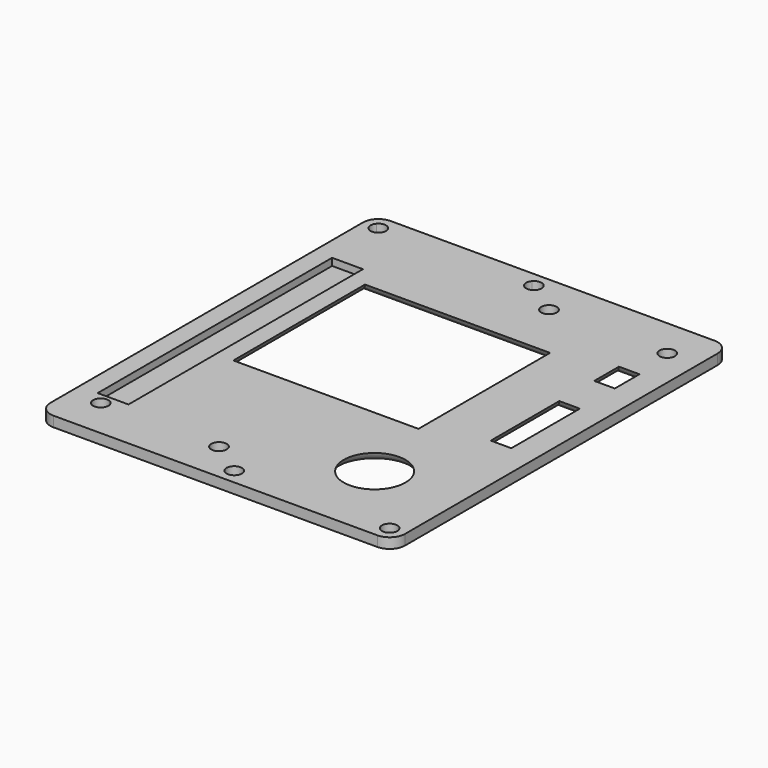
from build123d import *

# Parameters (mm, degrees)
F0_R          = 1.5
F0_R_2        = 6
F0_W          = 6
F0_H          = 57
F0_W_2        = 36
F0_H_2        = 32
F0_W_3        = 4
F0_H_3        = 16.6644380502
F0_H_4        = 6
F0_W_4        = 4.7
F0_H_5        = 2
F0_W_5        = 13
F0_W_6        = 2.3
F0_W_7        = 1.5
F0_W_8        = 9
F0_W_9        = 11
F1_DEPTH      = 2
F2_T1_DEPTH   = 16.6644380502
F2_T3_DEPTH   = 4
F2_T5_DEPTH   = 6
F2_T7_DEPTH   = 32
F2_T9_DEPTH   = 36
F2_T17_DEPTH  = 11.0710678119
F2_T21_DEPTH  = 23.7355058621
F2_T28_DEPTH  = 11.0710678119
F2_T32_DEPTH  = 23.7355058621
F2_T39_DEPTH  = 23.7355058621
F2_T43_DEPTH  = 11.0710678119
F2_T51_DEPTH  = 11.0710678119
F2_T56_DEPTH  = 23.7355058621
F2_T63_DEPTH  = 13.0710678119
F2_T67_DEPTH  = 11.0710678119
F2_T75_DEPTH  = 13.0710678119
F2_T79_DEPTH  = 11.0710678119
F2_T86_DEPTH  = 11.0710678119
F2_T91_DEPTH  = 13.0710678119
F2_S93_R      = 1.5
F2_T94_DEPTH  = 8
F2_T100_DEPTH = 13.0710678119
F2_T104_DEPTH = 11.0710678119
F2_T111_DEPTH = 43.0710678119
F2_T115_DEPTH = 39.0710678119
F2_T122_DEPTH = 39.0710678119
F2_T126_DEPTH = 43.0710678119
F2_T133_DEPTH = 39.0710678119
F2_T137_DEPTH = 43.0710678119
F2_T145_DEPTH = 39.0710678119
F2_T149_DEPTH = 43.0710678119
F3_R          = 3
F4_DEPTH      = 0.6


# Not quite as in the source:
# - a fillet or chamfer that OpenCascade refuses, or shapes differently, is made with other operations: its cross-section is extruded or revolved along the edge and cut away or added


with BuildPart() as f1:
    # F0 (on Top) → F1 (new body)
    with BuildSketch(Plane.XY):
        with BuildLine():
            Line((12.5, -41), (34.5, -41))
            Line((34.5, -41), (34.5, 39))
            Line((34.5, 39), (28.5, 39))
            Line((28.5, 39), (25.5, 39))
            Line((25.5, 39), (20.8, 39))
            Line((20.8, 39), (7.8, 39))
            Line((7.8, 39), (5.5, 39))
            Line((5.5, 39), (-0.1319660113, 39))
            ThreePointArc((-0.1319660113, 39), (0.1512585384, 38.5352331347), (0.25, 38))
            ThreePointArc((0.25, 38), (-1.7852331347, 36.5987414616), (-2.3680339887, 39))
            Line((-2.3680339887, 39), (-5.5, 39))
            Line((-5.5, 39), (-14.5, 39))
            Line((-14.5, 39), (-25.5, 39))
            Line((-25.5, 39), (-27, 39))
            Line((-27, 39), (-28.5, 39))
            Line((-28.5, 39), (-30.3819660113, 39))
            ThreePointArc((-30.3819660113, 39), (-30.0987414616, 38.5352331347), (-30, 38))
            ThreePointArc((-30, 38), (-32.0352331347, 36.5987414616), (-32.6180339887, 39))
            Line((-32.6180339887, 39), (-34.5, 39))
            Line((-34.5, 39), (-34.5, -41))
            Line((-34.5, -41), (-12.5, -41))
            Line((-12.5, -41), (-10.5, -41))
            Line((-10.5, -41), (10.5, -41))
            Line((10.5, -41), (12.5, -41))
        make_face()
        with Locations((-28.5, -33.25)):
            Circle(F0_R, mode=Mode.SUBTRACT)
        with Locations((-5.5, -33.25)):
            Circle(F0_R, mode=Mode.SUBTRACT)
        with Locations((1.25, -38)):
            Circle(F0_R, mode=Mode.SUBTRACT)
        with Locations((31.5, -38)):
            Circle(F0_R, mode=Mode.SUBTRACT)
        with Locations((18, -24.7891994715)):
            Circle(F0_R_2, mode=Mode.SUBTRACT)
        with Locations((-27.9, -2.5)):
            Rectangle(F0_W, F0_H, mode=Mode.SUBTRACT)
        with Locations((-3.5, 6.25)):
            Rectangle(F0_W_2, F0_H_2, mode=Mode.SUBTRACT)
        with Locations((-28.5, 33.25)):
            Circle(F0_R, mode=Mode.SUBTRACT)
        with Locations((-5.5, 33.25)):
            Circle(F0_R, mode=Mode.SUBTRACT)
        with Locations((27.5, 2.4177809749)):
            Rectangle(F0_W_3, F0_H_3, mode=Mode.SUBTRACT)
        with Locations((5.5, 33.25)):
            Circle(F0_R, mode=Mode.SUBTRACT)
        with Locations((27.5, 22.25)):
            Rectangle(F0_W_3, F0_H_4, mode=Mode.SUBTRACT)
        with Locations((28.5, 33.25)):
            Circle(F0_R, mode=Mode.SUBTRACT)
        Polygon((28.5, 39), (34.5, 39), (34.5, 41), (28, 41), (25.5, 41), (25.5, 39), align=None)
        with Locations((23.15, 40)):
            Rectangle(F0_W_4, F0_H_5)
        with Locations((14.3, 40)):
            Rectangle(F0_W_5, F0_H_5)
        with Locations((6.65, 40)):
            Rectangle(F0_W_6, F0_H_5)
        with BuildLine():
            Line((-34.5, 41), (-34.5, 39))
            Line((-34.5, 39), (-32.6180339887, 39))
            ThreePointArc((-32.6180339887, 39), (-31.5, 39.5), (-30.3819660113, 39))
            Line((-30.3819660113, 39), (-28.5, 39))
            Line((-28.5, 39), (-27, 39))
            Line((-27, 39), (-27, 41))
            Line((-27, 41), (-34.5, 41))
        make_face()
        with BuildLine():
            Line((-0.1319660113, 39), (5.5, 39))
            Line((5.5, 39), (5.5, 41))
            Line((5.5, 41), (-5.5, 41))
            Line((-5.5, 41), (-5.5, 39))
            Line((-5.5, 39), (-2.3680339887, 39))
            ThreePointArc((-2.3680339887, 39), (-1.25, 39.5), (-0.1319660113, 39))
        make_face()
        with Locations((-26.25, 40)):
            Rectangle(F0_W_7, F0_H_5)
        with Locations((-10, 40)):
            Rectangle(F0_W_8, F0_H_5)
        with Locations((-20, 40)):
            Rectangle(F0_W_9, F0_H_5)
        with Locations((-28.5, 33.25)):
            Circle(F0_R)
        with Locations((-5.5, 33.25)):
            Circle(F0_R)
    extrude(amount=F1_DEPTH)

    # F2: fillet of radius 3 on 13 edges, made by hand

    # F2_s2 → F2_t1 (cut)
    with BuildSketch(Plane.XZ.offset(-10.75)):
        with BuildLine():
            ThreePointArc((25.5, 2), (24.4036236828, 0.5505102572), (22.6715728753, 0))
            Line((22.6715728753, 0), (25.5, 0))
            Line((25.5, 0), (25.5, 2))
        make_face()
        with BuildLine():
            ThreePointArc((29.5, 2), (30.5963763172, 0.5505102572), (32.3284271247, 0))
            Line((32.3284271247, 0), (29.5, 0))
            Line((29.5, 0), (29.5, 2))
        make_face()
    extrude(amount=F2_T1_DEPTH, mode=Mode.SUBTRACT)

    # F2_s4 → F2_t3 (cut)
    with BuildSketch(Plane.YZ.offset(25.5)):
        with BuildLine():
            ThreePointArc((-5.9144380502, 2), (-7.0108143674, 0.5505102572), (-8.742865175, 0))
            Line((-8.742865175, 0), (-5.9144380502, 0))
            Line((-5.9144380502, 0), (-5.9144380502, 2))
        make_face()
        with BuildLine():
            ThreePointArc((10.75, 2), (11.8463763172, 0.5505102572), (13.5784271247, 0))
            Line((13.5784271247, 0), (10.75, 0))
            Line((10.75, 0), (10.75, 2))
        make_face()
        with BuildLine():
            ThreePointArc((19.25, 2), (18.1536236828, 0.5505102572), (16.4215728753, 0))
            Line((16.4215728753, 0), (19.25, 0))
            Line((19.25, 0), (19.25, 2))
        make_face()
        with BuildLine():
            ThreePointArc((25.25, 2), (26.3463763172, 0.5505102572), (28.0784271247, 0))
            Line((28.0784271247, 0), (25.25, 0))
            Line((25.25, 0), (25.25, 2))
        make_face()
    extrude(amount=F2_T3_DEPTH, mode=Mode.SUBTRACT)

    # F2_s6 → F2_t5 (cut)
    with BuildSketch(Plane.XZ.offset(-25.25)):
        with BuildLine():
            ThreePointArc((29.5, 2), (30.5963763172, 0.5505102572), (32.3284271247, 0))
            Line((32.3284271247, 0), (29.5, 0))
            Line((29.5, 0), (29.5, 2))
        make_face()
        with BuildLine():
            ThreePointArc((25.5, 2), (24.4036236828, 0.5505102572), (22.6715728753, 0))
            Line((22.6715728753, 0), (25.5, 0))
            Line((25.5, 0), (25.5, 2))
        make_face()
    extrude(amount=F2_T5_DEPTH, mode=Mode.SUBTRACT)

    # F2_s8 → F2_t7 (cut)
    with BuildSketch(Plane.XZ.offset(-22.25)):
        with BuildLine():
            ThreePointArc((14.5, 2), (15.5963763172, 0.5505102572), (17.3284271247, 0))
            Line((17.3284271247, 0), (14.5, 0))
            Line((14.5, 0), (14.5, 2))
        make_face()
        with BuildLine():
            ThreePointArc((-21.5, 2), (-22.5963763172, 0.5505102572), (-24.3284271247, 0))
            Line((-24.3284271247, 0), (-21.5, 0))
            Line((-21.5, 0), (-21.5, 2))
        make_face()
    extrude(amount=F2_T7_DEPTH, mode=Mode.SUBTRACT)

    # F2_s10 → F2_t9 (cut)
    with BuildSketch(Plane.YZ.offset(-21.5)):
        with BuildLine():
            ThreePointArc((-9.75, 2), (-10.8463763172, 0.5505102572), (-12.5784271247, 0))
            Line((-12.5784271247, 0), (-9.75, 0))
            Line((-9.75, 0), (-9.75, 2))
        make_face()
        with BuildLine():
            ThreePointArc((22.25, 2), (23.3463763172, 0.5505102572), (25.0784271247, 0))
            Line((25.0784271247, 0), (22.25, 0))
            Line((22.25, 0), (22.25, 2))
        make_face()
    extrude(amount=F2_T9_DEPTH, mode=Mode.SUBTRACT)

    # F2_s11 → F2_t12 (revolve, cut)
    with BuildSketch(Plane.XZ.offset(24.7891994715)):
        with BuildLine():
            ThreePointArc((24, 2), (25.0963763172, 0.5505102572), (26.8284271247, 0))
            Line((26.8284271247, 0), (24, 0))
            Line((24, 0), (24, 2))
        make_face()
    revolve(axis=Axis((18, -24.7891994715, 0), (0, 0, 1)), mode=Mode.SUBTRACT)


with BuildPart() as f2_tool15:
    # F2_s16 → F2_t17 (new body)
    with BuildSketch(Plane.YZ.offset(29.5)):
        with BuildLine():
            ThreePointArc((-5.9144380502, 2), (-7.0108143674, 0.5505102572), (-8.742865175, 0))
            Line((-8.742865175, 0), (-5.9144380502, 0))
            Line((-5.9144380502, 0), (-5.9144380502, 2))
        make_face()
    extrude(amount=-F2_T17_DEPTH)

    split(bisect_by=Plane.YZ.offset(25.5), keep=Keep.BOTTOM)


with BuildPart() as f2_tool19:
    # F2_s20 → F2_t21 (new body)
    with BuildSketch(Plane.XZ.offset(12.9855058621)):
        with BuildLine():
            ThreePointArc((25.5, 2), (24.4036236828, 0.5505102572), (22.6715728753, 0))
            Line((22.6715728753, 0), (25.5, 0))
            Line((25.5, 0), (25.5, 2))
        make_face()
    extrude(amount=-F2_T21_DEPTH)

    split(bisect_by=Plane.XZ.offset(5.9144380502), keep=Keep.TOP)


with BuildPart() as f2_tool15_1:
    add(f2_tool15.part)

    # F2_t23: intersect F2_tool19
    add(f2_tool19.part, mode=Mode.INTERSECT)


with BuildPart() as f1_1:
    add(f1.part)

    # F2_t13: cut F2_tool15
    add(f2_tool15_1.part, mode=Mode.SUBTRACT)


with BuildPart() as f2_tool26:
    # F2_s27 → F2_t28 (new body)
    with BuildSketch(Plane.YZ.offset(18.4289321881)):
        with BuildLine():
            ThreePointArc((10.75, 2), (11.8463763172, 0.5505102572), (13.5784271247, 0))
            Line((13.5784271247, 0), (10.75, 0))
            Line((10.75, 0), (10.75, 2))
        make_face()
    extrude(amount=F2_T28_DEPTH)

    split(bisect_by=Plane.YZ.offset(25.5), keep=Keep.BOTTOM)


with BuildPart() as f2_tool30:
    # F2_s31 → F2_t32 (new body)
    with BuildSketch(Plane.XZ.offset(5.9144380502)):
        with BuildLine():
            ThreePointArc((25.5, 2), (24.4036236828, 0.5505102572), (22.6715728753, 0))
            Line((22.6715728753, 0), (25.5, 0))
            Line((25.5, 0), (25.5, 2))
        make_face()
    extrude(amount=-F2_T32_DEPTH)

    split(bisect_by=Plane.XZ.offset(-10.75), keep=Keep.BOTTOM)


with BuildPart() as f2_tool26_1:
    add(f2_tool26.part)

    # F2_t34: intersect F2_tool30
    add(f2_tool30.part, mode=Mode.INTERSECT)


with BuildPart() as f1_2:
    add(f1_1.part)

    # F2_t24: cut F2_tool26
    add(f2_tool26_1.part, mode=Mode.SUBTRACT)


with BuildPart() as f2_tool37:
    # F2_s38 → F2_t39 (new body)
    with BuildSketch(Plane.XZ.offset(-10.75)):
        with BuildLine():
            ThreePointArc((29.5, 2), (30.5963763172, 0.5505102572), (32.3284271247, 0))
            Line((32.3284271247, 0), (29.5, 0))
            Line((29.5, 0), (29.5, 2))
        make_face()
    extrude(amount=F2_T39_DEPTH)

    split(bisect_by=Plane.XZ.offset(5.9144380502), keep=Keep.TOP)


with BuildPart() as f2_tool41:
    # F2_s42 → F2_t43 (new body)
    with BuildSketch(Plane.YZ.offset(36.5710678119)):
        with BuildLine():
            ThreePointArc((-5.9144380502, 2), (-7.0108143674, 0.5505102572), (-8.742865175, 0))
            Line((-8.742865175, 0), (-5.9144380502, 0))
            Line((-5.9144380502, 0), (-5.9144380502, 2))
        make_face()
    extrude(amount=-F2_T43_DEPTH)

    split(bisect_by=Plane.YZ.offset(34.5), keep=Keep.BOTTOM)

    split(bisect_by=Plane.YZ.offset(29.5), keep=Keep.TOP)


with BuildPart() as f2_tool37_1:
    add(f2_tool37.part)

    # F2_t46: intersect F2_tool41
    add(f2_tool41.part, mode=Mode.INTERSECT)


with BuildPart() as f1_3:
    add(f1_2.part)

    # F2_t35: cut F2_tool37
    add(f2_tool37_1.part, mode=Mode.SUBTRACT)


with BuildPart() as f2_tool49:
    # F2_s50 → F2_t51 (new body)
    with BuildSketch(Plane.YZ.offset(25.5)):
        with BuildLine():
            ThreePointArc((10.75, 2), (11.8463763172, 0.5505102572), (13.5784271247, 0))
            Line((13.5784271247, 0), (10.75, 0))
            Line((10.75, 0), (10.75, 2))
        make_face()
    extrude(amount=F2_T51_DEPTH)

    split(bisect_by=Plane.YZ.offset(34.5), keep=Keep.BOTTOM)

    split(bisect_by=Plane.YZ.offset(29.5), keep=Keep.TOP)


with BuildPart() as f2_tool54:
    # F2_s55 → F2_t56 (new body)
    with BuildSketch(Plane.XZ.offset(-17.8210678119)):
        with BuildLine():
            ThreePointArc((29.5, 2), (30.5963763172, 0.5505102572), (32.3284271247, 0))
            Line((32.3284271247, 0), (29.5, 0))
            Line((29.5, 0), (29.5, 2))
        make_face()
    extrude(amount=F2_T56_DEPTH)

    split(bisect_by=Plane.XZ.offset(-10.75), keep=Keep.BOTTOM)


with BuildPart() as f2_tool49_1:
    add(f2_tool49.part)

    # F2_t58: intersect F2_tool54
    add(f2_tool54.part, mode=Mode.INTERSECT)


with BuildPart() as f1_4:
    add(f1_3.part)

    # F2_t47: cut F2_tool49
    add(f2_tool49_1.part, mode=Mode.SUBTRACT)


with BuildPart() as f2_tool61:
    # F2_s62 → F2_t63 (new body)
    with BuildSketch(Plane.XZ.offset(-25.25)):
        with BuildLine():
            ThreePointArc((29.5, 2), (30.5963763172, 0.5505102572), (32.3284271247, 0))
            Line((32.3284271247, 0), (29.5, 0))
            Line((29.5, 0), (29.5, 2))
        make_face()
    extrude(amount=F2_T63_DEPTH)

    split(bisect_by=Plane.XZ.offset(-19.25), keep=Keep.TOP)


with BuildPart() as f2_tool65:
    # F2_s66 → F2_t67 (new body)
    with BuildSketch(Plane.YZ.offset(36.5710678119)):
        with BuildLine():
            ThreePointArc((19.25, 2), (18.1536236828, 0.5505102572), (16.4215728753, 0))
            Line((16.4215728753, 0), (19.25, 0))
            Line((19.25, 0), (19.25, 2))
        make_face()
    extrude(amount=-F2_T67_DEPTH)

    split(bisect_by=Plane.YZ.offset(34.5), keep=Keep.BOTTOM)

    split(bisect_by=Plane.YZ.offset(29.5), keep=Keep.TOP)


with BuildPart() as f2_tool61_1:
    add(f2_tool61.part)

    # F2_t70: intersect F2_tool65
    add(f2_tool65.part, mode=Mode.INTERSECT)


with BuildPart() as f1_5:
    add(f1_4.part)

    # F2_t59: cut F2_tool61
    add(f2_tool61_1.part, mode=Mode.SUBTRACT)


with BuildPart() as f2_tool73:
    # F2_s74 → F2_t75 (new body)
    with BuildSketch(Plane.XZ.offset(-12.1789321881)):
        with BuildLine():
            ThreePointArc((25.5, 2), (24.4036236828, 0.5505102572), (22.6715728753, 0))
            Line((22.6715728753, 0), (25.5, 0))
            Line((25.5, 0), (25.5, 2))
        make_face()
    extrude(amount=-F2_T75_DEPTH)

    split(bisect_by=Plane.XZ.offset(-19.25), keep=Keep.TOP)


with BuildPart() as f2_tool77:
    # F2_s78 → F2_t79 (new body)
    with BuildSketch(Plane.YZ.offset(29.5)):
        with BuildLine():
            ThreePointArc((19.25, 2), (18.1536236828, 0.5505102572), (16.4215728753, 0))
            Line((16.4215728753, 0), (19.25, 0))
            Line((19.25, 0), (19.25, 2))
        make_face()
    extrude(amount=-F2_T79_DEPTH)

    split(bisect_by=Plane.YZ.offset(25.5), keep=Keep.BOTTOM)


with BuildPart() as f2_tool73_1:
    add(f2_tool73.part)

    # F2_t81: intersect F2_tool77
    add(f2_tool77.part, mode=Mode.INTERSECT)


with BuildPart() as f1_6:
    add(f1_5.part)

    # F2_t71: cut F2_tool73
    add(f2_tool73_1.part, mode=Mode.SUBTRACT)


with BuildPart() as f2_tool84:
    # F2_s85 → F2_t86 (new body)
    with BuildSketch(Plane.YZ.offset(25.5)):
        with BuildLine():
            ThreePointArc((25.25, 2), (26.3463763172, 0.5505102572), (28.0784271247, 0))
            Line((28.0784271247, 0), (25.25, 0))
            Line((25.25, 0), (25.25, 2))
        make_face()
    extrude(amount=F2_T86_DEPTH)

    split(bisect_by=Plane.YZ.offset(34.5), keep=Keep.BOTTOM)

    split(bisect_by=Plane.YZ.offset(29.5), keep=Keep.TOP)


with BuildPart() as f2_tool89:
    # F2_s90 → F2_t91 (new body)
    with BuildSketch(Plane.XZ.offset(-32.3210678119)):
        with BuildLine():
            ThreePointArc((29.5, 2), (30.5963763172, 0.5505102572), (32.3284271247, 0))
            Line((32.3284271247, 0), (29.5, 0))
            Line((29.5, 0), (29.5, 2))
        make_face()
    extrude(amount=F2_T91_DEPTH)

    split(bisect_by=Plane.XZ.offset(-25.25), keep=Keep.BOTTOM)

    # F2_s93 → F2_t94 (cut, symmetric)
    with BuildSketch(Plane.XY.offset(1)):
        with Locations((28.5, 33.25)):
            Circle(F2_S93_R)
    extrude(amount=F2_T94_DEPTH, both=True, mode=Mode.SUBTRACT)


with BuildPart() as f2_tool84_1:
    add(f2_tool84.part)

    # F2_t95: intersect F2_tool89
    add(f2_tool89.part, mode=Mode.INTERSECT)


with BuildPart() as f1_7:
    add(f1_6.part)

    # F2_t82: cut F2_tool84
    add(f2_tool84_1.part, mode=Mode.SUBTRACT)


with BuildPart() as f2_tool98:
    # F2_s99 → F2_t100 (new body)
    with BuildSketch(Plane.XZ.offset(-19.25)):
        with BuildLine():
            ThreePointArc((25.5, 2), (24.4036236828, 0.5505102572), (22.6715728753, 0))
            Line((22.6715728753, 0), (25.5, 0))
            Line((25.5, 0), (25.5, 2))
        make_face()
    extrude(amount=-F2_T100_DEPTH)

    split(bisect_by=Plane.XZ.offset(-25.25), keep=Keep.BOTTOM)


with BuildPart() as f2_tool102:
    # F2_s103 → F2_t104 (new body)
    with BuildSketch(Plane.YZ.offset(18.4289321881)):
        with BuildLine():
            ThreePointArc((25.25, 2), (26.3463763172, 0.5505102572), (28.0784271247, 0))
            Line((28.0784271247, 0), (25.25, 0))
            Line((25.25, 0), (25.25, 2))
        make_face()
    extrude(amount=F2_T104_DEPTH)

    split(bisect_by=Plane.YZ.offset(25.5), keep=Keep.BOTTOM)


with BuildPart() as f2_tool98_1:
    add(f2_tool98.part)

    # F2_t106: intersect F2_tool102
    add(f2_tool102.part, mode=Mode.INTERSECT)


with BuildPart() as f1_8:
    add(f1_7.part)

    # F2_t96: cut F2_tool98
    add(f2_tool98_1.part, mode=Mode.SUBTRACT)


with BuildPart() as f2_tool109:
    # F2_s110 → F2_t111 (new body)
    with BuildSketch(Plane.YZ.offset(-21.5)):
        with BuildLine():
            ThreePointArc((22.25, 2), (23.3463763172, 0.5505102572), (25.0784271247, 0))
            Line((25.0784271247, 0), (22.25, 0))
            Line((22.25, 0), (22.25, 2))
        make_face()
    extrude(amount=F2_T111_DEPTH)

    split(bisect_by=Plane.YZ.offset(14.5), keep=Keep.TOP)


with BuildPart() as f2_tool113:
    # F2_s114 → F2_t115 (new body)
    with BuildSketch(Plane.XZ.offset(-29.3210678119)):
        with BuildLine():
            ThreePointArc((14.5, 2), (15.5963763172, 0.5505102572), (17.3284271247, 0))
            Line((17.3284271247, 0), (14.5, 0))
            Line((14.5, 0), (14.5, 2))
        make_face()
    extrude(amount=F2_T115_DEPTH)

    split(bisect_by=Plane.XZ.offset(-22.25), keep=Keep.BOTTOM)


with BuildPart() as f2_tool109_1:
    add(f2_tool109.part)

    # F2_t117: intersect F2_tool113
    add(f2_tool113.part, mode=Mode.INTERSECT)


with BuildPart() as f1_9:
    add(f1_8.part)

    # F2_t107: cut F2_tool109
    add(f2_tool109_1.part, mode=Mode.SUBTRACT)


with BuildPart() as f2_tool120:
    # F2_s121 → F2_t122 (new body)
    with BuildSketch(Plane.XZ.offset(-22.25)):
        with BuildLine():
            ThreePointArc((14.5, 2), (15.5963763172, 0.5505102572), (17.3284271247, 0))
            Line((17.3284271247, 0), (14.5, 0))
            Line((14.5, 0), (14.5, 2))
        make_face()
    extrude(amount=F2_T122_DEPTH)

    split(bisect_by=Plane.XZ.offset(9.75), keep=Keep.TOP)


with BuildPart() as f2_tool124:
    # F2_s125 → F2_t126 (new body)
    with BuildSketch(Plane.YZ.offset(21.5710678119)):
        with BuildLine():
            ThreePointArc((-9.75, 2), (-10.8463763172, 0.5505102572), (-12.5784271247, 0))
            Line((-12.5784271247, 0), (-9.75, 0))
            Line((-9.75, 0), (-9.75, 2))
        make_face()
    extrude(amount=-F2_T126_DEPTH)

    split(bisect_by=Plane.YZ.offset(14.5), keep=Keep.TOP)


with BuildPart() as f2_tool120_1:
    add(f2_tool120.part)

    # F2_t128: intersect F2_tool124
    add(f2_tool124.part, mode=Mode.INTERSECT)


with BuildPart() as f1_10:
    add(f1_9.part)

    # F2_t118: cut F2_tool120
    add(f2_tool120_1.part, mode=Mode.SUBTRACT)


with BuildPart() as f2_tool131:
    # F2_s132 → F2_t133 (new body)
    with BuildSketch(Plane.XZ.offset(16.8210678119)):
        with BuildLine():
            ThreePointArc((-21.5, 2), (-22.5963763172, 0.5505102572), (-24.3284271247, 0))
            Line((-24.3284271247, 0), (-21.5, 0))
            Line((-21.5, 0), (-21.5, 2))
        make_face()
    extrude(amount=-F2_T133_DEPTH)

    split(bisect_by=Plane.XZ.offset(9.75), keep=Keep.TOP)


with BuildPart() as f2_tool135:
    # F2_s136 → F2_t137 (new body)
    with BuildSketch(Plane.YZ.offset(14.5)):
        with BuildLine():
            ThreePointArc((-9.75, 2), (-10.8463763172, 0.5505102572), (-12.5784271247, 0))
            Line((-12.5784271247, 0), (-9.75, 0))
            Line((-9.75, 0), (-9.75, 2))
        make_face()
    extrude(amount=-F2_T137_DEPTH)

    split(bisect_by=Plane.YZ.offset(-24.9), keep=Keep.TOP)

    split(bisect_by=Plane.YZ.offset(-21.5), keep=Keep.BOTTOM)


with BuildPart() as f2_tool131_1:
    add(f2_tool131.part)

    # F2_t140: intersect F2_tool135
    add(f2_tool135.part, mode=Mode.INTERSECT)


with BuildPart() as f1_11:
    add(f1_10.part)

    # F2_t129: cut F2_tool131
    add(f2_tool131_1.part, mode=Mode.SUBTRACT)


with BuildPart() as f2_tool143:
    # F2_s144 → F2_t145 (new body)
    with BuildSketch(Plane.XZ.offset(9.75)):
        with BuildLine():
            ThreePointArc((-21.5, 2), (-22.5963763172, 0.5505102572), (-24.3284271247, 0))
            Line((-24.3284271247, 0), (-21.5, 0))
            Line((-21.5, 0), (-21.5, 2))
        make_face()
    extrude(amount=-F2_T145_DEPTH)

    split(bisect_by=Plane.XZ.offset(-22.25), keep=Keep.BOTTOM)


with BuildPart() as f2_tool147:
    # F2_s148 → F2_t149 (new body)
    with BuildSketch(Plane.YZ.offset(-28.5710678119)):
        with BuildLine():
            ThreePointArc((22.25, 2), (23.3463763172, 0.5505102572), (25.0784271247, 0))
            Line((25.0784271247, 0), (22.25, 0))
            Line((22.25, 0), (22.25, 2))
        make_face()
    extrude(amount=F2_T149_DEPTH)

    split(bisect_by=Plane.YZ.offset(-24.9), keep=Keep.TOP)

    split(bisect_by=Plane.YZ.offset(-21.5), keep=Keep.BOTTOM)


with BuildPart() as f2_tool143_1:
    add(f2_tool143.part)

    # F2_t152: intersect F2_tool147
    add(f2_tool147.part, mode=Mode.INTERSECT)


with BuildPart() as f1_12:
    add(f1_11.part)

    # F2_t141: cut F2_tool143
    add(f2_tool143_1.part, mode=Mode.SUBTRACT)

    # F3
    f3_edges = [f1_12.edges().sort_by_distance(p)[0] for p in [
        (-34.5, 41, 1),
        (34.5, 41, 1),
        (34.5, -41, 1),
        (-34.5, -41, 1),
    ]]
    fillet(f3_edges, radius=F3_R)

    # F0 (on Top) → F4 (join)
    with BuildSketch(Plane.XY):
        with Locations((-27.9, -2.5)):
            Rectangle(F0_W, F0_H)
    extrude(amount=F4_DEPTH)


solid = f1_12.part
